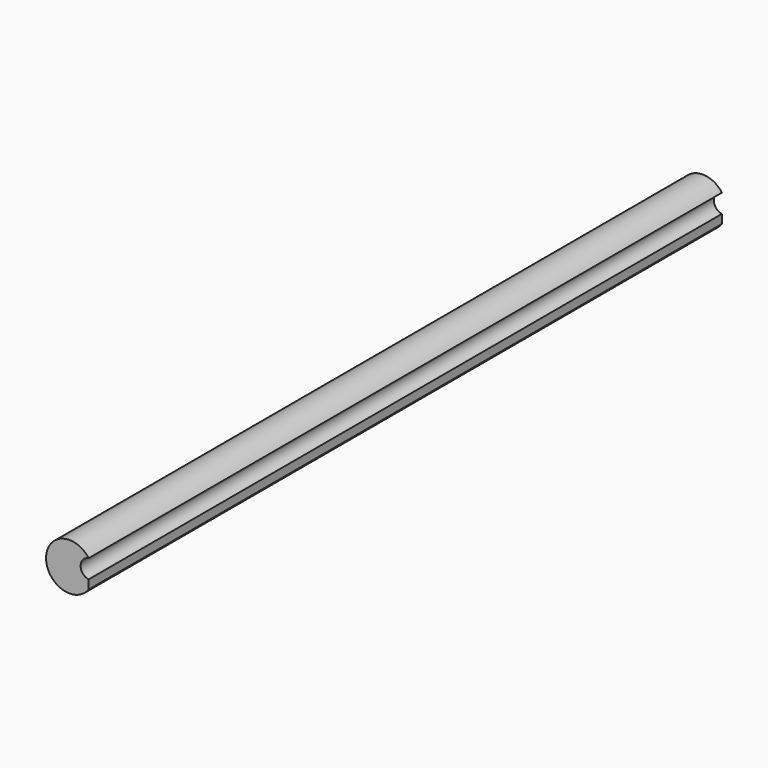
from build123d import *

# Parameters (mm, degrees)
F1_DEPTH = 8368.7720298767


with BuildPart() as f1:
    # F0 (on Front) → F1 (new body)
    with BuildSketch(Plane.XZ):
        with BuildLine():
            ThreePointArc((-76.8094025219, -30.2340624724), (-161.2325249757, 69.1179944594), (-75.9702353455, 167.7508327458))
            ThreePointArc((-75.9702353455, 167.7508327459), (-526.9220006184, 22.800048198), (-76.5748455344, -124.0184262918))
            ThreePointArc((-76.5748455344, -124.0184262918), (-77.095014232, -77.1272520204), (-76.8094025219, -30.2340624724))
        make_face()
    extrude(amount=F1_DEPTH)


solid = f1.part
